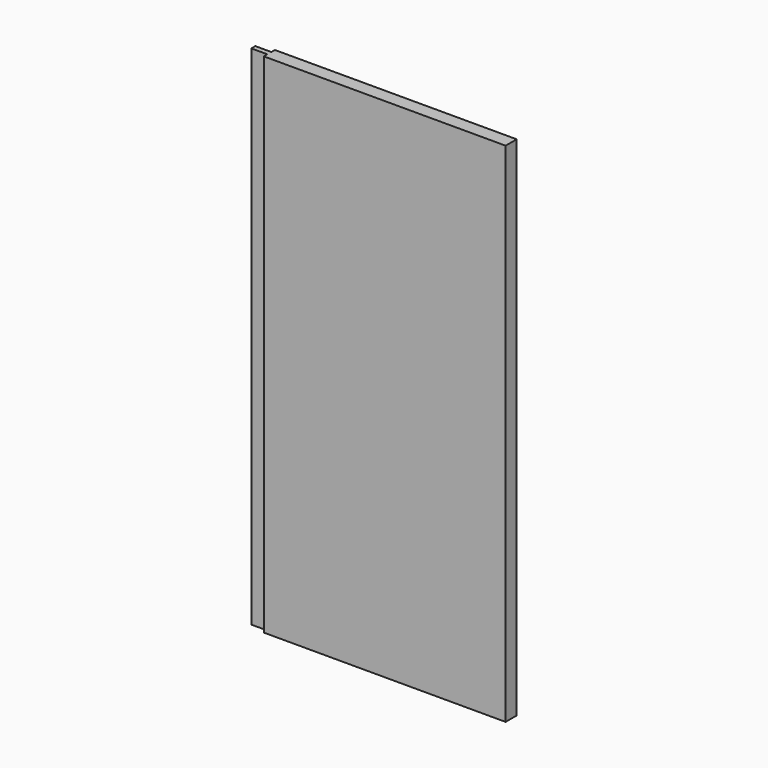
from build123d import *

# Parameters (mm, degrees)
F0_W     = 43.6125099659
F0_H     = 91.5184393525
F1_DEPTH = 2.5
F2_W     = 0.9
F2_H     = 91.5184393525
F3_DEPTH = 2.9


# Not quite as in the source:
# - a feature of the source that left no trace in its solid (it failed there, or was rolled back) is left out


with BuildPart() as f1:
    # F0 (on Front) → F1 (new body)
    with BuildSketch(Plane.XZ):
        with Locations((-21.8062549829, 0)):
            Rectangle(F0_W, F0_H)
    extrude(amount=-F1_DEPTH)

    # F2 (on face) → F3 (join)
    with BuildSketch(Plane(origin=(-43.6125099659, 0, 0), x_dir=(0, -1, 0), z_dir=(-1, 0, 0))):
        with Locations((-1.25, 0)):
            Rectangle(F2_W, F2_H)
    extrude(amount=F3_DEPTH)


solid = f1.part
